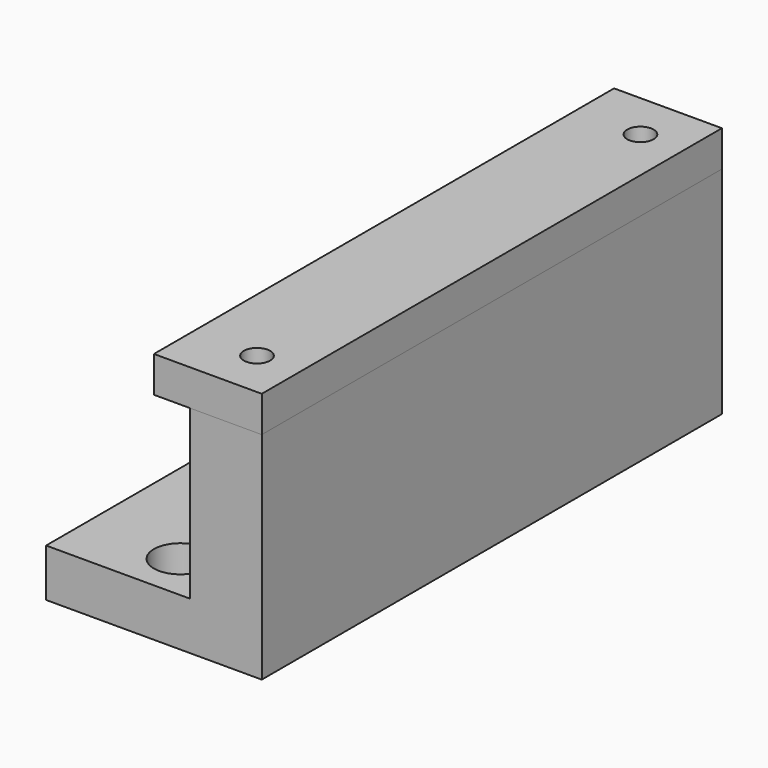
from build123d import *

# Parameters (mm, degrees)
F1_DEPTH = 240
F3_D     = 22
F5_D     = 10.3
F5_DEPTH = 20
F5_TIP   = 3.094432188
F6_W     = 45
F6_H     = 240
F7_DEPTH = 15
F8_D     = 11


# Not quite as in the source:
# - a feature names something its author has since deleted; it is built from what else it names


with BuildPart() as f1:
    # F0 (on Front) → F1 (new body)
    with BuildSketch(Plane.XZ):
        Polygon((-30, 20), (-90, 20), (-90, 0), (0, 0), (0, 90), (-30, 90), align=None)
    extrude(amount=-F1_DEPTH)

    # F3 (through all)
    with Locations(Plane.XY.offset(20)):
        with Locations((-50, 220), (-50, 20), (-50, 220), (-50, 20)):
            Hole(F3_D / 2)

    # F5
    with Locations(Plane.XY.offset(90)):
        with Locations((-18, 220), (-18, 20)):
            Hole(F5_D / 2, depth=F5_DEPTH)
            with Locations((0, 0, -(F5_DEPTH + F5_TIP / 2))):  # 118° drill point
                Cone(0, F5_D / 2, F5_TIP, mode=Mode.SUBTRACT)


with BuildPart() as f7:
    # F6 (on face) → F7 (new body)
    with BuildSketch(Plane.XY.offset(90)):
        with Locations((-22.5, 120)):
            Rectangle(F6_W, F6_H)
    extrude(amount=F7_DEPTH)

    # F8 (through all)
    with Locations(Plane(origin=(0, 0, 90), x_dir=(1, 0, 0), z_dir=(0, 0, -1))):
        with Locations((-18, -220), (-18, -20)):
            Hole(F8_D / 2)


solid = Compound([f1.part, f7.part])
